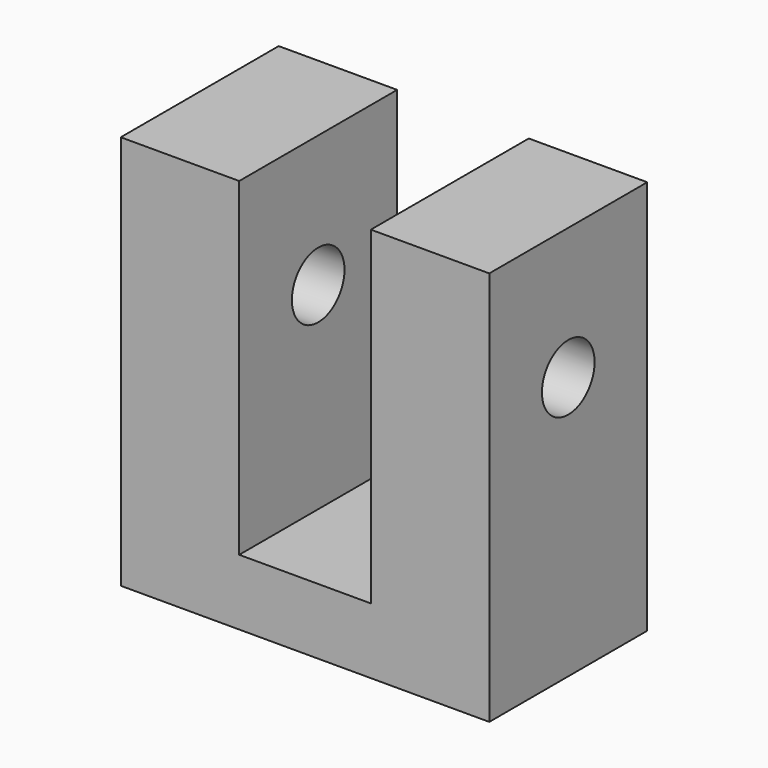
from build123d import *

# Parameters (mm, degrees)
F0_W     = 1.4
F0_H     = 1.5
F1_DEPTH = 0.75
F2_R     = 0.125
F3_DEPTH = 12.5
F4_R     = 0.125
F5_DEPTH = 0.5
F6_W     = 0.5
F6_H     = 1.25
F7_DEPTH = 25


# Not quite as in the source:
# - a feature names something its author has since deleted; it is built from what else it names


with BuildPart() as f1:
    # F0 (on Front) → F1 (new body)
    with BuildSketch(Plane.XZ):
        Rectangle(F0_W, F0_H)
    extrude(amount=F1_DEPTH)

    # F2 (on Right) → F3 (cut, symmetric)
    with BuildSketch(Plane.YZ):
        with Locations((-0.375, 0.25)):
            Circle(F2_R)
    extrude(amount=F3_DEPTH, both=True, mode=Mode.SUBTRACT)

    # F4 (on face) → F5 (cut)
    with BuildSketch(Plane(origin=(0, 0, -0.75), x_dir=(1, 0, 0), z_dir=(0, 0, -1))):
        with Locations((0.512, 0.5)):
            Circle(F4_R)
        with Locations((-0.512, 0.5)):
            Circle(F4_R)
    extrude(amount=-F5_DEPTH, mode=Mode.SUBTRACT)

    # F6 (on face) → F7 (cut)
    with BuildSketch(Plane.XZ.offset(0.75)):
        with Locations((0, 0.125)):
            Rectangle(F6_W, F6_H)
    extrude(amount=-F7_DEPTH, mode=Mode.SUBTRACT)


solid = f1.part
